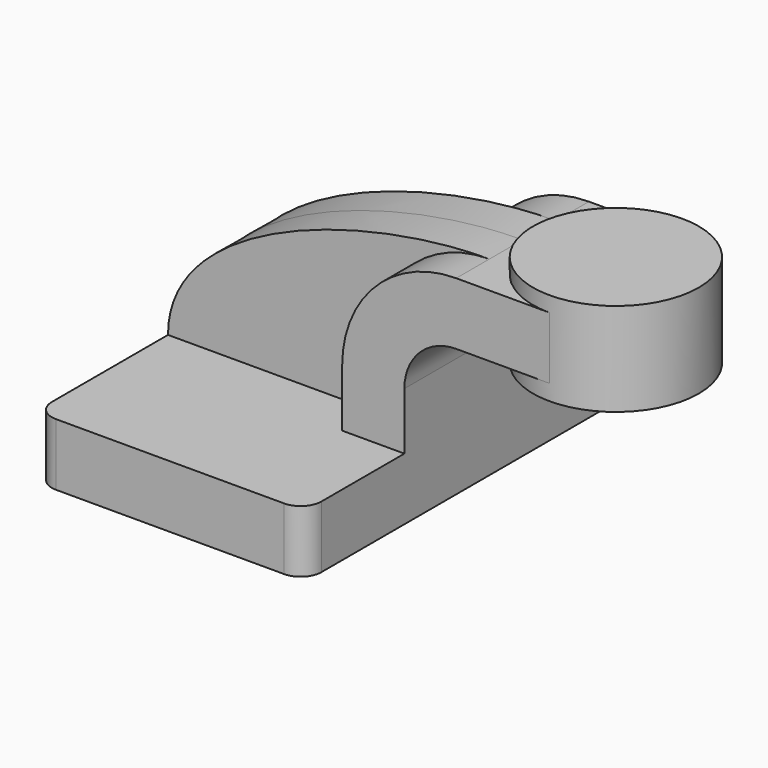
from build123d import *

# Parameters (mm, degrees)
F1_DEPTH = 63.5
F2_DEPTH = 25.4
F3_DEPTH = 12.7
F5_R     = 6.35


with BuildPart() as f1:
    # F0 (on Front) → F1 (new body, symmetric)
    with BuildSketch(Plane.XZ):
        Polygon((-41.275, 9.525), (-41.275, -9.525), (41.275, -9.525), (41.275, 9.525), (22.225, 9.525), align=None)
    extrude(amount=F1_DEPTH, both=True)

    # F0 (on Front) → F2 (join, symmetric)
    with BuildSketch(Plane.XZ):
        with BuildLine():
            Line((22.225, 9.525), (41.275, 9.525))
            Line((41.275, 9.525), (41.275, 27.051))
            ThreePointArc((41.275, 27.051), (45.9246798487, 38.2763201513), (57.15, 42.926))
            Line((57.15, 42.926), (60.325, 42.926))
            Line((60.325, 42.926), (60.325, 61.976))
            Line((60.325, 61.976), (57.15, 61.976))
            ThreePointArc((57.15, 61.976), (32.4542956671, 51.7467043329), (22.225, 27.051))
            Line((22.225, 27.051), (22.225, 9.525))
        make_face()
        Polygon((82.0737038128, 61.976), (60.325, 61.976), (60.325, 42.926), (82.0737038128, 42.926), (85.725, 42.926), (85.725, 61.976), align=None)
    extrude(amount=F2_DEPTH, both=True)

    # F0 (on Front) → F3 (join, symmetric)
    with BuildSketch(Plane.XZ):
        with BuildLine():
            add(Edge.make_bspline(
                [(-41.275, 9.525), (-41.2416942418, 43.5823909938), (19.5547696203, 62.110837549), (57.15, 61.976)],
                knots=[0, 0, 0, 0, 111.5284180198, 111.5284180198, 111.5284180198, 111.5284180198], degree=3))
            Line((-41.275, 9.525), (22.225, 9.525))
            Line((22.225, 9.525), (22.225, 27.051))
            ThreePointArc((22.225, 27.051), (32.4542956671, 51.7467043329), (57.15, 61.976))
        make_face()
    extrude(amount=F3_DEPTH, both=True)

    # F0 (on Front) → F4 (revolve)
    with BuildSketch(Plane.XZ):
        Polygon((111.125, 66.675), (85.725, 66.675), (85.725, 61.976), (85.725, 42.926), (85.725, 38.1), (111.125, 38.1), align=None)
    revolve(axis=Axis((85.725, 0, 52.3875), (0, 0, 1)))

    # F5
    f5_edges = [f1.edges().sort_by_distance(p)[0] for p in [
        (-41.275, -63.5, 0),
        (41.275, -63.5, 0),
        (41.275, 63.5, 0),
        (-41.275, 63.5, 0),
    ]]
    fillet(f5_edges, radius=F5_R)


solid = f1.part
